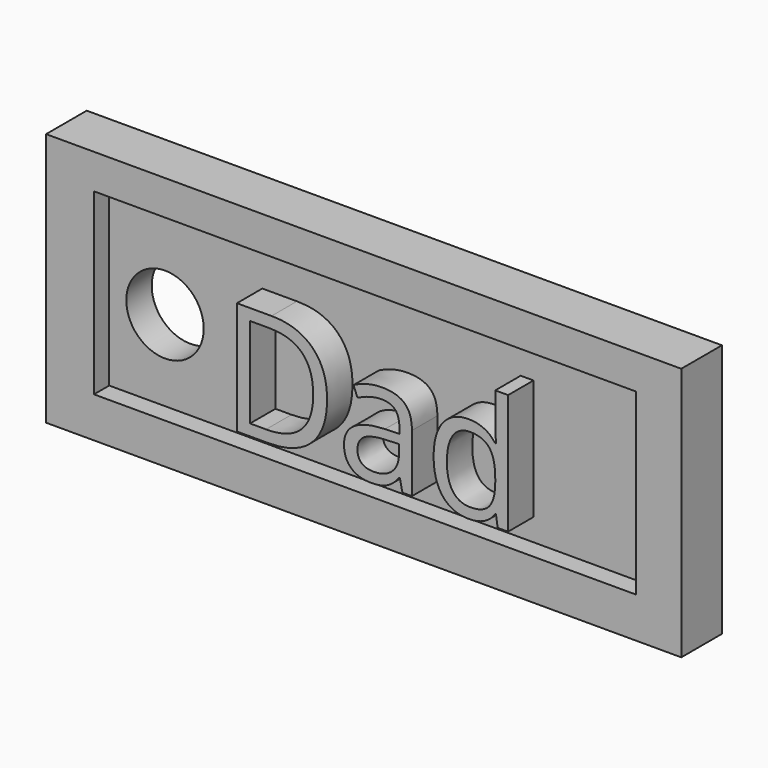
from build123d import *

# Parameters (mm, degrees)
F0_W         = 63.5
F0_H         = 25.4
F0_W_2       = 54.169384297
F0_H_2       = 17.8703125566
F1_DEPTH     = 5.08
F2_DEPTH     = 3.175
F4_TEXT_SIZE = 15.8170632656
F5_DEPTH     = 6.35
F3_R         = 3.870606587
F6_DEPTH     = 25.4


# Not quite as in the source:
# - Text() gives the source's letters only with a copy of the font that has no kerning and outlines rounded to 1/6400 em; it was checked with that copy


with BuildPart() as f1:
    # F0 (on Front) → F1 (new body)
    with BuildSketch(Plane.XZ):
        with Locations((31.75, 12.7)):
            Rectangle(F0_W, F0_H)
        with Locations((31.8721954245, 12.9888067022)):
            Rectangle(F0_W_2, F0_H_2, mode=Mode.SUBTRACT)
    extrude(amount=F1_DEPTH)

    # F0 (on Front) → F2 (join)
    with BuildSketch(Plane.XZ):
        with Locations((31.8721954245, 12.9888067022)):
            Rectangle(F0_W_2, F0_H_2)
    extrude(amount=F2_DEPTH)

    # F4 (on Front) → F5 (join)
    with BuildSketch(Plane.XZ):
        with Locations((18.5424648225, 6.2781567685)):
            Text('Dad', F4_TEXT_SIZE, font='Open Sans', text_align=(TextAlign.LEFT, TextAlign.BOTTOM))
    extrude(amount=F5_DEPTH)

    # F3 (on face) → F6 (cut)
    with BuildSketch(Plane.XZ.offset(3.175)):
        with Locations((10.3662591428, 12.118303217)):
            Circle(F3_R)
    extrude(amount=-F6_DEPTH, mode=Mode.SUBTRACT)


solid = f1.part
